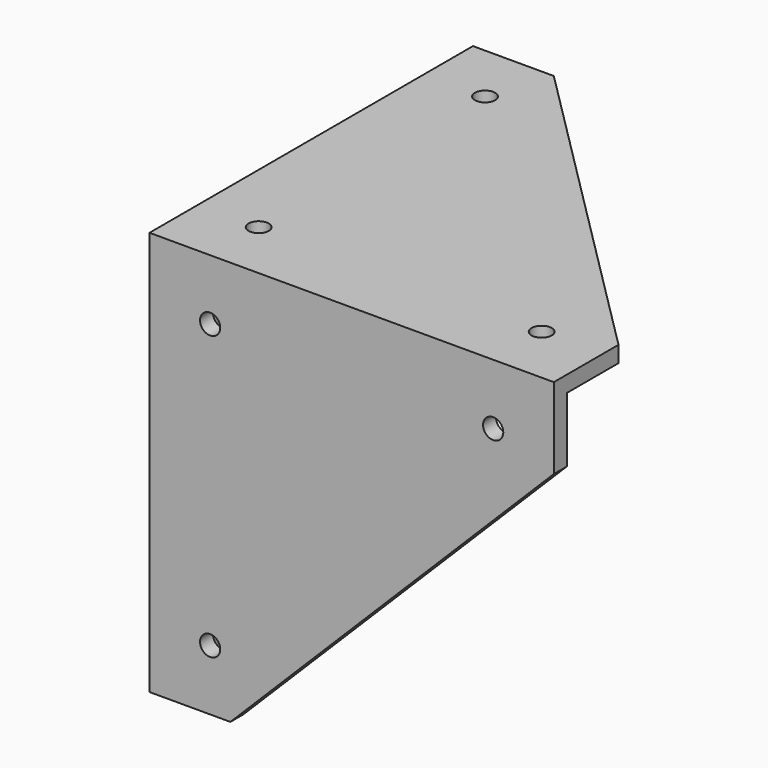
from build123d import *

# Parameters (mm, degrees)
F1_DEPTH  = 4
F4_DEPTH  = 4
F9_DEPTH  = 4
F10_R     = 2
F11_DEPTH = 4
F12_R     = 2.5
F13_DEPTH = 4
F14_R     = 2.5
F15_DEPTH = 4
F16_R     = 2.5
F17_DEPTH = 4


with BuildPart() as f1:
    # F0 (on Top) → F1 (new body)
    with BuildSketch(Plane.XY):
        Polygon((-28.663731938, 61.6347389425), (-48.663731938, 61.6347389425), (-48.663731938, -38.3652610575), (51.336268062, -38.3652610575), (51.336268062, -18.3652610575), align=None)
    extrude(amount=F1_DEPTH)



with BuildPart() as f4:
    # F3 (on offset) → F4 (new body)
    with BuildSketch(Plane(origin=(-48.663731938, 0, 0), x_dir=(0, -1, 0), z_dir=(-1, 0, 0))):
        Polygon((38.3652610575, 0), (-61.6347389425, 0), (-61.6347389425, -20), (14.3654177458, -95.9132762154), (38.3652610575, -96), align=None)
    extrude(amount=-F4_DEPTH)


with BuildPart() as f1_1:
    add(f1.part)

    add(f4.part)  # F9 merges F4
    # F8 (on offset) → F9 (join)
    with BuildSketch(Plane.XZ.offset(38.3652610575)):
        Polygon((51.336268062, -16), (51.336268062, 4), (-48.663731938, 4), (-48.663731938, -96), (-28.663731938, -96), align=None)
    extrude(amount=-F9_DEPTH)

    # F10 (on face) → F11 (cut)
    with BuildSketch(Plane.XZ.offset(38.3652610575)):
        with Locations((36.336268062, -11)):
            Circle(F10_R)
        with Locations((-33.663731938, -11)):
            Circle(F10_R)
        with Locations((-33.663731938, -81)):
            Circle(F10_R)
    extrude(amount=-F11_DEPTH, mode=Mode.SUBTRACT)

    # F12 (on face) → F13 (cut)
    with BuildSketch(Plane.XZ.offset(38.3652610575)):
        with Locations((36.336268062, -11)):
            Circle(F12_R)
        with Locations((-33.663731938, -11)):
            Circle(F12_R)
        with Locations((-33.663731938, -81)):
            Circle(F12_R)
    extrude(amount=-F13_DEPTH, mode=Mode.SUBTRACT)

    # F14 (on face) → F15 (cut)
    with BuildSketch(Plane(origin=(-48.663731938, 0, 0), x_dir=(0, -1, 0), z_dir=(-1, 0, 0))):
        with Locations((-46.6681093954, -11)):
            Circle(F14_R)
        with Locations((20.8652610575, -11)):
            Circle(F14_R)
        with Locations((23.3652610575, -80.9456993499)):
            Circle(F14_R)
    extrude(amount=-F15_DEPTH, mode=Mode.SUBTRACT)

    # F16 (on face) → F17 (cut)
    with BuildSketch(Plane.XY.offset(4)):
        with Locations((-33.663731938, 46.6347389425)):
            Circle(F16_R)
        with Locations((-33.663731938, -23.3652610575)):
            Circle(F16_R)
        with Locations((36.336268062, -23.3652610575)):
            Circle(F16_R)
    extrude(amount=-F17_DEPTH, mode=Mode.SUBTRACT)


solid = f1_1.part
